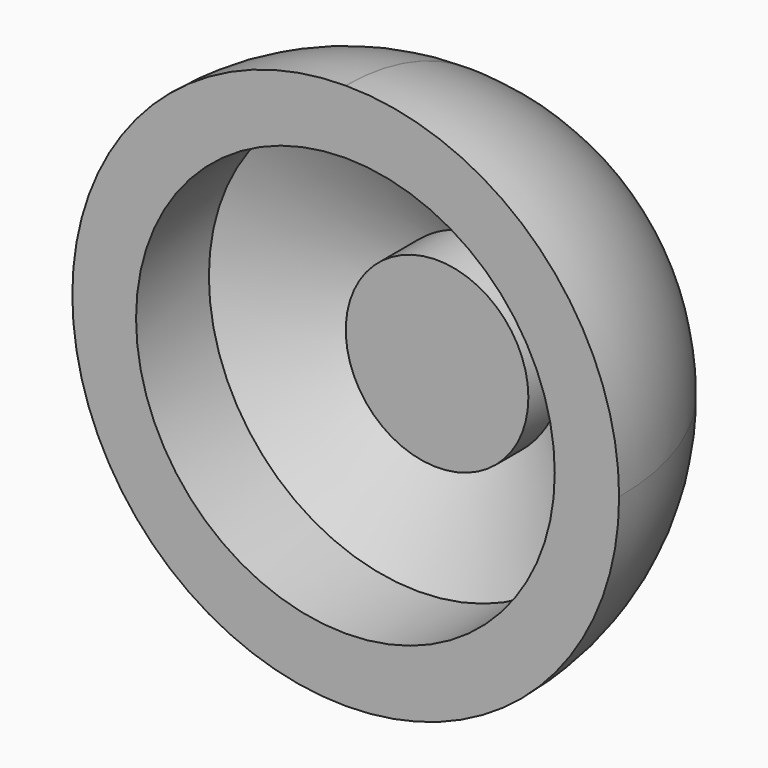
from build123d import *

# Parameters (mm, degrees)
F0_W     = 76.2886069715
F0_H     = 38.1443016231
F1_DEPTH = 76.2
F2_R     = 38.09999
F4_D     = 58.42
F4_DEPTH = 12.7
F4_TIP   = 17.5511386818
F5_R     = 38.09999
F6_R     = 12.7378189323
F7_DEPTH = 25.4


# Not quite as in the source:
# - a fillet or chamfer is up to 0.001 mm smaller than in the source, because OpenCascade refuses the exact size


with BuildPart() as f1:
    # F0 (on Top) → F1 (new body)
    with BuildSketch(Plane.XY):
        with Locations((-1.0466407984, 2.4421662092)):
            Rectangle(F0_W, F0_H)
    extrude(amount=F1_DEPTH)

    # F2 (radius 38.1 in the source; OpenCascade refuses exactly that, so slightly less here)
    f2_edges = [f1.edges().sort_by_distance(p)[0] for p in [
        (-39.190944, 2.442166, 76.2),
        (-39.190944, 2.442166, 0),
        (37.097663, 2.442166, 76.2),
        (37.097663, 2.442166, 0),
    ]]
    fillet(f2_edges, radius=F2_R)

    # F4
    with Locations(Plane.XZ.offset(16.6299846023)):
        with Locations((-1.0909442842, 38.1)):
            Hole(F4_D / 2, depth=F4_DEPTH)
            with Locations((0, 0, -(F4_DEPTH + F4_TIP / 2))):  # 118° drill point
                Cone(0, F4_D / 2, F4_TIP, mode=Mode.SUBTRACT)

    # F5 (radius 38.1 in the source; OpenCascade refuses exactly that, so slightly less here)
    f5_edges = [f1.edges().sort_by_distance(p)[0] for p in [
        (-28.031716, 21.514317, 11.159229),
        (25.938434, 21.514317, 11.159229),
    ]]
    fillet(f5_edges, radius=F5_R)

    # F6 (on Front) → F7 (join)
    with BuildSketch(Plane.XZ):
        with Locations((-1.6050767154, 35.1008698344)):
            Circle(F6_R)
    extrude(amount=-F7_DEPTH)


solid = f1.part
